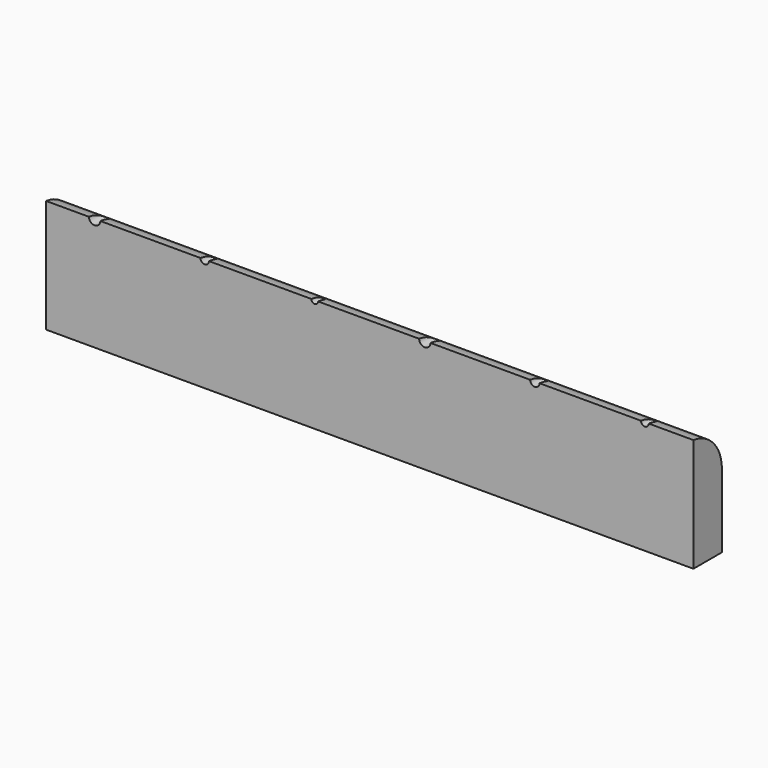
from build123d import *

# Parameters (mm, degrees)
F0_W        = 50.8
F0_H        = 2.794
F1_DEPTH    = 8.89
F2_T1_DEPTH = 66.5602855304
F4_DEPTH    = 25.4


# Not quite as in the source:
# - a fillet or chamfer that OpenCascade refuses, or shapes differently, is made with other operations: its cross-section is extruded or revolved along the edge and cut away or added


with BuildPart() as f1:
    # F0 (on Top) → F1 (new body)
    with BuildSketch(Plane.XY):
        with Locations((0, 1.397)):
            Rectangle(F0_W, F0_H)
    extrude(amount=F1_DEPTH)

    # F2: fillet of radius 3.175 on 1 edges, made by hand

    # F2_s2 → F2_t1 (cut)
    with BuildSketch(Plane.YZ.offset(-33.2801427652)):
        with BuildLine():
            ThreePointArc((2.794, 5.7379428939), (1.9949524406, 7.8439996358), (0, 8.89))
            Line((0, 8.89), (2.794, 8.89))
            Line((2.794, 8.89), (2.794, 5.7379428939))
        make_face()
    extrude(amount=F2_T1_DEPTH, mode=Mode.SUBTRACT)

    # F3 (on face) → F4 (cut)
    with BuildSketch(Plane.XZ):
        with BuildLine():
            ThreePointArc((-22.0345, 8.89), (-21.59, 8.4455), (-21.1455, 8.89))
            Line((-21.1455, 8.89), (-22.0345, 8.89))
        make_face()
        with BuildLine():
            Line((-12.6238, 8.89), (-13.2842, 8.89))
            ThreePointArc((-13.2842, 8.89), (-12.954, 8.5598), (-12.6238, 8.89))
        make_face()
        with BuildLine():
            Line((13.3223, 8.89), (12.5857, 8.89))
            ThreePointArc((12.5857, 8.89), (12.954, 8.5217), (13.3223, 8.89))
        make_face()
        with BuildLine():
            ThreePointArc((21.2852, 8.89), (21.59, 8.5852), (21.8948, 8.89))
            Line((21.8948, 8.89), (21.2852, 8.89))
        make_face()
        with BuildLine():
            Line((-4.0513, 8.89), (-4.5847, 8.89))
            ThreePointArc((-4.5847, 8.89), (-4.318, 8.6233), (-4.0513, 8.89))
        make_face()
        with BuildLine():
            Line((4.7625, 8.89), (3.8735, 8.89))
            ThreePointArc((3.8735, 8.89), (4.318, 8.4455), (4.7625, 8.89))
        make_face()
    extrude(amount=-F4_DEPTH, mode=Mode.SUBTRACT)


solid = f1.part
